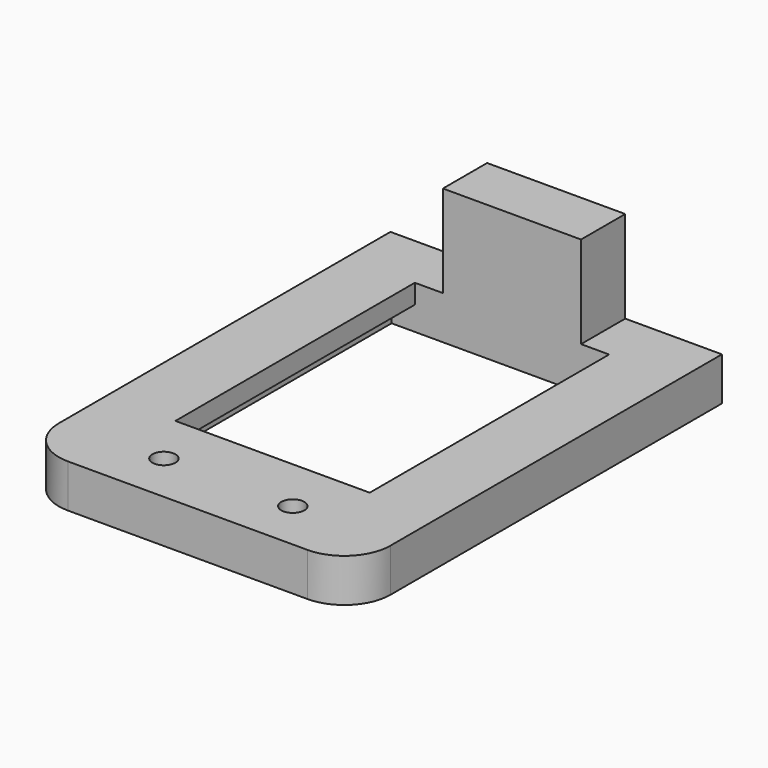
from build123d import *

# Parameters (mm, degrees)
F0_W     = 72
F0_H     = 100
F1_DEPTH = 9.4
F2_W     = 42.2
F2_H     = 65
F3_DEPTH = 5.2
F4_DEPTH = 9.4
F5_W     = 30
F5_H     = 12
F6_DEPTH = 20
F7_R     = 2.5
F8_DEPTH = 9.4
F9_R     = 10


# Not quite as in the source:
# - a feature names something its author has since deleted; it is built from what else it names


with BuildPart() as f1:
    # F0 (on Top) → F1 (new body)
    with BuildSketch(Plane.XY):
        Rectangle(F0_W, F0_H)
    extrude(amount=F1_DEPTH)

    # F2 (on face) → F3 (cut)
    with BuildSketch(Plane(origin=(0, 0, 0), x_dir=(1, 0, 0), z_dir=(0, 0, -1))):
        Polygon((21.1, -38), (26.15, -38), (26.15, 37), (-26.15, 37), (-26.15, -38), (-21.1, -38), (-21.1, 27), (21.1, 27), align=None)
        with Locations((0, -5.5)):
            Rectangle(F2_W, F2_H)
    extrude(amount=-F3_DEPTH, mode=Mode.SUBTRACT)

    # F2 (on face) → F4 (cut, through all)
    with BuildSketch(Plane(origin=(0, 0, 0), x_dir=(1, 0, 0), z_dir=(0, 0, -1))):
        with Locations((0, -5.5)):
            Rectangle(F2_W, F2_H)
    extrude(amount=-F4_DEPTH, mode=Mode.SUBTRACT)

    # F5 (on face) → F6 (join)
    with BuildSketch(Plane.XY.offset(9.4)):
        with Locations((0, 44)):
            Rectangle(F5_W, F5_H)
    extrude(amount=F6_DEPTH)

    # F7 (on face) → F8 (cut, through all)
    with BuildSketch(Plane.XY.offset(9.4)):
        with Locations((-14, -39)):
            Circle(F7_R)
        with Locations((14, -39)):
            Circle(F7_R)
    extrude(amount=-F8_DEPTH, mode=Mode.SUBTRACT)

    # F9
    f9_edges = [f1.edges().sort_by_distance(p)[0] for p in [
        (36, -50, 4.7),
        (-36, -50, 4.7),
    ]]
    fillet(f9_edges, radius=F9_R)


solid = f1.part
